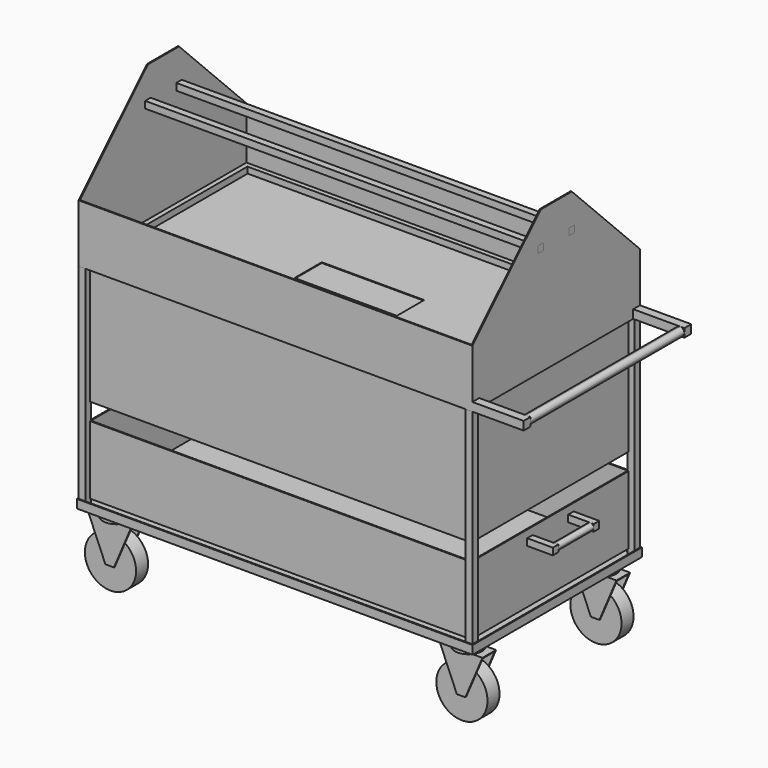
from build123d import *

# Parameters (mm, degrees)
F0_W      = 1120
F0_H      = 580
F1_DEPTH  = 350
F2_DEPTH  = 250
F3_DEPTH  = 50
F4_T      = -3
F5_W      = 1160
F5_H      = 620
F5_W_2    = 1120
F5_H_2    = 580
F6_DEPTH  = 25
F7_T      = -3
F8_W      = 20
F8_H      = 20.8832610362
F9_DEPTH  = 622
F8_H_2    = 20
F10_T     = -2.5
F10_2_T   = -2.5
F10_3_T   = -2.5
F10_4_T   = -2.5
F11_W     = 1154
F11_H     = 614
F11_W_2   = 1120
F11_H_2   = 580
F12_DEPTH = 20
F13_W     = 3
F13_H     = 614
F14_DEPTH = 400
F16_DEPTH = 1160
F17_W     = 20
F17_H     = 20
F18_DEPTH = 1153
F19_W     = 1148
F19_H     = 3
F20_DEPTH = 20
F21_W     = 20
F21_H     = 20
F22_DEPTH = 75
F24_DEPTH = 140
F25_W     = 25
F25_H     = 25
F26_DEPTH = 150
F28_DEPTH = 580
F29_R     = 40
F30_DEPTH = 25
F32_DEPTH = 3
F33_W     = 125
F33_H     = 3
F34_DEPTH = 115
F36_DEPTH = 50
F38_DEPTH = 44
F45_DEPTH = 2
F47_DEPTH = 130
F48_W     = 300
F48_H     = 100
F49_DEPTH = 3


with BuildPart() as f1:
    # F0 (on Top) → F1 (new body)
    with BuildSketch(Plane.XY):
        Rectangle(F0_W, F0_H)
    extrude(amount=F1_DEPTH)


with BuildPart() as f2:
    # F0 (on Top) → F2 (new body)
    with BuildSketch(Plane.XY):
        Rectangle(F0_W, F0_H)
    extrude(amount=-F2_DEPTH)

    # F0 (on Top) → F3 (cut)
    with BuildSketch(Plane.XY):
        Rectangle(F0_W, F0_H)
    extrude(amount=-F3_DEPTH, mode=Mode.SUBTRACT)

    # F4
    f4_openings = [f2.faces().sort_by_distance(p)[0] for p in [
        (0, 0, -50),
    ]]
    offset(amount=F4_T, openings=f4_openings)

    # F21 (on face) → F22 (join)
    with BuildSketch(Plane.YZ.offset(560)):
        with Locations((-75, -82.1892789321)):
            Rectangle(F21_W, F21_H)
        with Locations((75, -82.1892789321)):
            Rectangle(F21_W, F21_H)
    extrude(amount=F22_DEPTH)

    # F23 (on face) → F24 (join)
    with BuildSketch(Plane.XZ.offset(-65)):
        with BuildLine():
            ThreePointArc((625, -92.1892789321), (632.0710678119, -89.260346744), (635, -82.1892789321))
            ThreePointArc((635, -82.1892789321), (632.0710678119, -75.1182111203), (625, -72.1892789321))
            ThreePointArc((625, -72.1892789321), (615, -82.1892789321), (625, -92.1892789321))
        make_face()
    extrude(amount=F24_DEPTH)


with BuildPart() as f6:
    # F5 (on face) → F6 (new body)
    with BuildSketch(Plane(origin=(0, 0, -250), x_dir=(1, 0, 0), z_dir=(0, 0, -1))):
        Rectangle(F5_W, F5_H)
        Rectangle(F5_W_2, F5_H_2, mode=Mode.SUBTRACT)
        Rectangle(F5_W_2, F5_H_2)
    extrude(amount=F6_DEPTH)

    # F7
    f7_openings = [f6.faces().sort_by_distance(p)[0] for p in [
        (0, 0, -250),
    ]]
    offset(amount=F7_T, openings=f7_openings)


with BuildPart() as f9:
    # F8 (on face) → F9 (new body)
    with BuildSketch(Plane.XY.offset(-272)):
        with Locations((-567, 296.5583694819)):
            Rectangle(F8_W, F8_H)
    extrude(amount=F9_DEPTH)

    # F10
    f10_openings = [f9.faces().sort_by_distance(p)[0] for p in [
        (-567, 296.558369, 350),
    ]]
    offset(amount=F10_T, openings=f10_openings)


with BuildPart() as f9b:
    # F8 (on face) → F9, piece 2 (new body)
    with BuildSketch(Plane.XY.offset(-272)):
        with Locations((-567, -297)):
            Rectangle(F8_W, F8_H_2)
    extrude(amount=F9_DEPTH)

    # F10#4
    f10_4_openings = [f9b.faces().sort_by_distance(p)[0] for p in [
        (-567, -297, 350),
    ]]
    offset(amount=F10_4_T, openings=f10_4_openings)


with BuildPart() as f9c:
    # F8 (on face) → F9, piece 3 (new body)
    with BuildSketch(Plane.XY.offset(-272)):
        with Locations((567, 297)):
            Rectangle(F8_W, F8_H_2)
    extrude(amount=F9_DEPTH)

    # F10#2
    f10_2_openings = [f9c.faces().sort_by_distance(p)[0] for p in [
        (567, 297, 350),
    ]]
    offset(amount=F10_2_T, openings=f10_2_openings)


with BuildPart() as f9d:
    # F8 (on face) → F9, piece 4 (new body)
    with BuildSketch(Plane.XY.offset(-272)):
        with Locations((567, -297)):
            Rectangle(F8_W, F8_H_2)
    extrude(amount=F9_DEPTH)

    # F10#3
    f10_3_openings = [f9d.faces().sort_by_distance(p)[0] for p in [
        (567, -297, 350),
    ]]
    offset(amount=F10_3_T, openings=f10_3_openings)


with BuildPart() as f12:
    # F11 (on face) → F12 (new body)
    with BuildSketch(Plane.XY.offset(350)):
        Rectangle(F11_W, F11_H)
        Rectangle(F11_W_2, F11_H_2, mode=Mode.SUBTRACT)
    extrude(amount=F12_DEPTH)

    # F13 (on face) → F14 (join)
    with BuildSketch(Plane.XY.offset(370)):
        with Locations((575.5, 0)):
            Rectangle(F13_W, F13_H)
        with Locations((-575.5, 0)):
            Rectangle(F13_W, F13_H)
    extrude(amount=F14_DEPTH)

    # F15 (on face) → F16 (cut)
    with BuildSketch(Plane.YZ.offset(577)):
        Polygon((-57, 770), (-307, 770), (-307, 520), align=None)
        Polygon((307, 770), (57, 770), (307, 520), align=None)
    extrude(amount=-F16_DEPTH, mode=Mode.SUBTRACT)

    # F19 (on face) → F20 (join)
    with BuildSketch(Plane.XY.offset(370)):
        with Locations((0, -305.5)):
            Rectangle(F19_W, F19_H)
        with Locations((0, 305.5)):
            Rectangle(F19_W, F19_H)
    extrude(amount=F20_DEPTH)

    # F25 (on face) → F26 (join)
    with BuildSketch(Plane.YZ.offset(577)):
        with Locations((-294.5, 362.5)):
            Rectangle(F25_W, F25_H)
        with Locations((294.5, 362.5)):
            Rectangle(F25_W, F25_H)
    extrude(amount=F26_DEPTH)

    # F27 (on face) → F28 (join)
    with BuildSketch(Plane.XZ.offset(-282)):
        with BuildLine():
            ThreePointArc((714.5, 350), (723.3388347648, 353.6611652352), (727, 362.5))
            ThreePointArc((727, 362.5), (723.3388347648, 371.3388347648), (714.5, 375))
            ThreePointArc((714.5, 375), (702, 362.5), (714.5, 350))
        make_face()
    extrude(amount=F28_DEPTH)

    # F47 (add): faces of the model
    f47_faces = [f12.faces().sort_by_distance(p)[0] for p in [
        (0, -305.5, 390),
        (0, 305.5, 390),
    ]]
    extrude(f47_faces, amount=F47_DEPTH)


with BuildPart() as f18:
    # F17 (on face) → F18 (new body)
    with BuildSketch(Plane.YZ.offset(577)):
        with Locations((-57, 670)):
            Rectangle(F17_W, F17_H)
    extrude(amount=-F18_DEPTH)


with BuildPart() as f18b:
    # F17 (on face) → F18, piece 2 (new body)
    with BuildSketch(Plane.YZ.offset(577)):
        with Locations((57, 670)):
            Rectangle(F17_W, F17_H)
    extrude(amount=-F18_DEPTH)


with BuildPart() as f30:
    # F29 (on face) → F30 (new body)
    with BuildSketch(Plane(origin=(0, 0, -275), x_dir=(1, 0, 0), z_dir=(0, 0, -1))):
        with Locations((-515.4019242525, 245.4019242525)):
            Circle(F29_R)
    extrude(amount=F30_DEPTH)


with BuildPart() as f30b:
    # F29 (on face) → F30, piece 2 (new body)
    with BuildSketch(Plane(origin=(0, 0, -275), x_dir=(1, 0, 0), z_dir=(0, 0, -1))):
        with Locations((516.1099678278, 245.4019242525)):
            Circle(F29_R)
    extrude(amount=F30_DEPTH)


with BuildPart() as f30c:
    # F29 (on face) → F30, piece 3 (new body)
    with BuildSketch(Plane(origin=(0, 0, -275), x_dir=(1, 0, 0), z_dir=(0, 0, -1))):
        with Locations((516.1099678278, -246.1099678278)):
            Circle(F29_R)
    extrude(amount=F30_DEPTH)


with BuildPart() as f30d:
    # F29 (on face) → F30, piece 4 (new body)
    with BuildSketch(Plane(origin=(0, 0, -275), x_dir=(1, 0, 0), z_dir=(0, 0, -1))):
        with Locations((-515.4019242525, -246.1099678278)):
            Circle(F29_R)
    extrude(amount=F30_DEPTH)


with BuildPart() as f32:
    # F31 (on face) → F32 (new body)
    with BuildSketch(Plane(origin=(0, 0, -300), x_dir=(1, 0, 0), z_dir=(0, 0, -1))):
        with BuildLine():
            Line((-452.9019242525, 220.4019242525), (-452.9019242525, 270.4019242525))
            Line((-452.9019242525, 270.4019242525), (-484.1769342605, 270.4019242525))
            ThreePointArc((-484.1769342605, 270.4019242525), (-477.6593779706, 258.6495731066), (-475.4019242525, 245.4019242525))
            ThreePointArc((-475.4019242525, 245.4019242525), (-477.6593779706, 232.1542753985), (-484.1769342605, 220.4019242525))
            Line((-484.1769342605, 220.4019242525), (-452.9019242525, 220.4019242525))
        make_face()
        with BuildLine():
            ThreePointArc((-475.4019242525, 245.4019242525), (-477.6593779706, 258.6495731066), (-484.1769342605, 270.4019242525))
            Line((-484.1769342605, 270.4019242525), (-546.6269142445, 270.4019242525))
            ThreePointArc((-546.6269142445, 270.4019242525), (-555.4019242525, 245.4019242525), (-546.6269142445, 220.4019242525))
            Line((-546.6269142445, 220.4019242525), (-484.1769342605, 220.4019242525))
            ThreePointArc((-484.1769342605, 220.4019242525), (-477.6593779706, 232.1542753985), (-475.4019242525, 245.4019242525))
        make_face()
        with BuildLine():
            ThreePointArc((-546.6269142445, 220.4019242525), (-555.4019242525, 245.4019242525), (-546.6269142445, 270.4019242525))
            Line((-546.6269142445, 270.4019242525), (-577.9019242525, 270.4019242525))
            Line((-577.9019242525, 270.4019242525), (-577.9019242525, 220.4019242525))
            Line((-577.9019242525, 220.4019242525), (-546.6269142445, 220.4019242525))
        make_face()
    extrude(amount=F32_DEPTH)

    # F33 (on face) → F34 (join)
    with BuildSketch(Plane(origin=(0, 0, -303), x_dir=(1, 0, 0), z_dir=(0, 0, -1))):
        with Locations((-515.4019242525, 268.9019242525)):
            Rectangle(F33_W, F33_H)
        with Locations((-515.4019242525, 221.9019242525)):
            Rectangle(F33_W, F33_H)
    extrude(amount=F34_DEPTH)

    # F35 (on face) → F36 (cut)
    with BuildSketch(Plane(origin=(0, -220.4019242525, 0), x_dir=(-1, 0, 0), z_dir=(0, 1, 0))):
        Polygon((577.9019242525, -300), (527.9019242525, -418), (577.9019242525, -418), align=None)
        Polygon((452.9019242525, -418), (502.9019242525, -418), (452.9019242525, -300), align=None)
    extrude(amount=-F36_DEPTH, mode=Mode.SUBTRACT)


with BuildPart() as f38:
    # F37 (on face) → F38 (new body)
    with BuildSketch(Plane(origin=(0, -267.4019242525, 0), x_dir=(-1, 0, 0), z_dir=(0, 1, 0))):
        with BuildLine():
            ThreePointArc((472.5755318844, -346.4297140113), (480.6670673189, -474.4717211587), (590.4019242525, -408))
            ThreePointArc((590.4019242525, -408), (581.8736454112, -373.2651430664), (558.2283166206, -346.4297140113))
            Line((558.2283166206, -346.4297140113), (527.9019242525, -418))
            Line((527.9019242525, -418), (502.9019242525, -418))
            Line((502.9019242525, -418), (472.5755318844, -346.4297140113))
        make_face()
        with BuildLine():
            Line((527.9019242525, -418), (558.2283166206, -346.4297140113))
            ThreePointArc((558.2283166206, -346.4297140113), (515.4019242525, -333), (472.5755318844, -346.4297140113))
            Line((472.5755318844, -346.4297140113), (502.9019242525, -418))
            Line((502.9019242525, -418), (527.9019242525, -418))
        make_face()
    extrude(amount=F38_DEPTH)


with BuildPart() as f39_1:
    # F39: copy of F38
    add(f38.part.moved(Location((0, 491, 0))))


with BuildPart() as f40_1:
    # F40: copy of F32
    add(f32.part.moved(Location((0, 491, 0))))


with BuildPart() as f41_1:
    # F41: copy of F39_1
    add(f39_1.part.moved(Location((1030, 0, 0))))


with BuildPart() as f42_1:
    # F42: copy of F40_1
    add(f40_1.part.moved(Location((1030, 0, 0))))


with BuildPart() as f43_1:
    # F43: copy of F32
    add(f32.part.moved(Location((1030, 0, 0))))


with BuildPart() as f44_1:
    # F44: copy of F38
    add(f38.part.moved(Location((1030, 0, 0))))


with BuildPart() as f45:
    # F45 (new): a face of the model
    f45_faces = [f2.part.faces().sort_by_distance(p)[0] for p in [
        (0, 0, -247),
    ]]
    extrude(f45_faces, amount=F45_DEPTH)


with BuildPart() as f45_1:
    # F46: moved
    add(f45.part.moved(Location((0, 0, 599))))

    # F48 (on face) → F49 (cut)
    with BuildSketch(Plane.XY.offset(354)):
        Rectangle(F48_W, F48_H)
    extrude(amount=-F49_DEPTH, mode=Mode.SUBTRACT)


solid = Compound([f1.part, f2.part, f6.part, f9.part, f9b.part, f9c.part, f9d.part, f12.part, f18.part, f18b.part, f30.part, f30b.part, f30c.part, f30d.part, f32.part, f38.part, f39_1.part, f40_1.part, f41_1.part, f42_1.part, f43_1.part, f44_1.part, f45_1.part])
